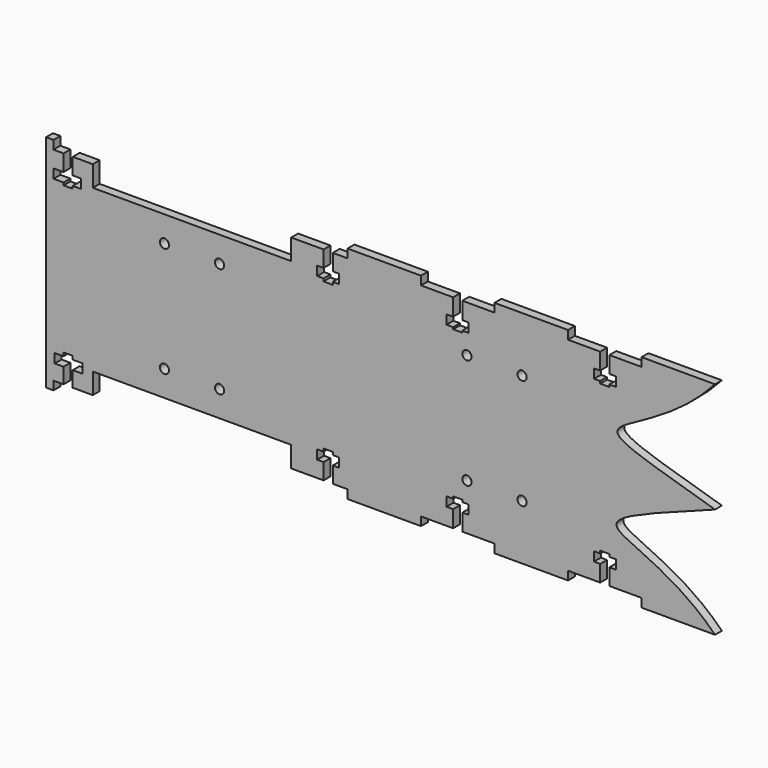
from build123d import *

# Parameters (mm, degrees)
F0_R     = 1.5875
F0_W     = 159.1020785272
F0_H     = 25.4
F1_DEPTH = 2.9718


# Not quite as in the source:
# - a feature names something its author has since deleted; it is built from what else it names


with BuildPart() as f1:
    # F0 (on Front) → F1 (new body)
    with BuildSketch(Plane.XZ):
        Polygon((-134.1324669933, 51.0296365122), (-134.1324669933, 54.0014365122), (-136.6724669933, 54.0014365122), (-136.6724669933, -22.1985634878), (-134.1324669933, -22.1985634878), (-134.1324669933, -19.2267634878), align=None)
        with BuildLine():
            Line((-130.6399669933, 51.0296365122), (-134.1324669933, 51.0296365122))
            Line((-134.1324669933, 51.0296365122), (-134.1324669933, -19.2267634878))
            Line((-134.1324669933, -19.2267634878), (-130.6399669933, -19.2267634878))
            Line((-130.6399669933, -19.2267634878), (-130.6399669933, -13.8642910361))
            Line((-130.6399669933, -13.8642910361), (-133.683725667, -13.8642910361))
            Line((-133.683725667, -13.8642910361), (-133.683725667, -10.6892910361))
            Line((-133.683725667, -10.6892910361), (-130.6399669933, -10.6892910361))
            Line((-130.6399669933, -10.6892910361), (-130.6399669933, -9.4985634878))
            Line((-130.6399669933, -9.4985634878), (-127.4649669933, -9.4985634878))
            Line((-127.4649669933, -9.4985634878), (-127.4649669933, -10.6892910361))
            Line((-127.4649669933, -10.6892910361), (-124.158725667, -10.6892910361))
            Line((-124.158725667, -10.6892910361), (-124.158725667, -13.8642910361))
            Line((-124.158725667, -13.8642910361), (-127.4649669933, -13.8642910361))
            Line((-127.4649669933, -13.8642910361), (-127.4649669933, -19.2267634878))
            Line((-127.4649669933, -19.2267634878), (-120.5434669933, -19.2267634878))
            Line((-120.5434669933, -19.2267634878), (-120.5434669933, -12.0385634878))
            Line((-120.5434669933, -12.0385634878), (-51.9634669933, -12.0385634878))
            Line((-51.9634669933, -12.0385634878), (-51.9634669933, -19.2267634878))
            Line((-51.9634669933, -19.2267634878), (-40.7874669933, -19.2267634878))
            Line((-40.7874669933, -19.2267634878), (-40.7874669933, -13.650716418))
            Line((-40.7874669933, -13.650716418), (-43.0311936414, -13.650716418))
            Line((-43.0311936414, -13.650716418), (-43.0311936414, -10.475716418))
            Line((-43.0311936414, -10.475716418), (-40.7874669933, -10.475716418))
            Line((-40.7874669933, -10.475716418), (-40.7874669933, -9.4985634878))
            Line((-40.7874669933, -9.4985634878), (-37.6124669933, -9.4985634878))
            Line((-37.6124669933, -9.4985634878), (-37.6124669933, -10.475716418))
            Line((-37.6124669933, -10.475716418), (-35.4111936414, -10.475716418))
            Line((-35.4111936414, -10.475716418), (-35.4111936414, -13.650716418))
            Line((-35.4111936414, -13.650716418), (-37.6124669933, -13.650716418))
            Line((-37.6124669933, -13.650716418), (-37.6124669933, -19.2267634878))
            Line((-37.6124669933, -19.2267634878), (-32.5324669933, -19.2267634878))
            Line((-32.5324669933, -19.2267634878), (-32.5324669933, -22.1985634878))
            Line((-32.5324669933, -22.1985634878), (-7.1324669933, -22.1985634878))
            Line((-7.1324669933, -22.1985634878), (-7.1324669933, -19.2267634878))
            Line((-7.1324669933, -19.2267634878), (3.9800330067, -19.2267634878))
            Line((3.9800330067, -19.2267634878), (3.9800330067, -13.4051909164))
            Line((3.9800330067, -13.4051909164), (1.6932926612, -13.4051909164))
            Line((1.6932926612, -13.4051909164), (1.6932926612, -10.2301909164))
            Line((1.6932926612, -10.2301909164), (3.9800330067, -10.2301909164))
            Line((3.9800330067, -10.2301909164), (3.9800330067, -9.4985634878))
            Line((3.9800330067, -9.4985634878), (7.1550330067, -9.4985634878))
            Line((7.1550330067, -9.4985634878), (7.1550330067, -10.2301909164))
            Line((7.1550330067, -10.2301909164), (9.3132926612, -10.2301909164))
            Line((9.3132926612, -10.2301909164), (9.3132926612, -13.4051909164))
            Line((9.3132926612, -13.4051909164), (7.1550330067, -13.4051909164))
            Line((7.1550330067, -13.4051909164), (7.1550330067, -19.2267634878))
            Line((7.1550330067, -19.2267634878), (18.2675330067, -19.2267634878))
            Line((18.2675330067, -19.2267634878), (18.2675330067, -22.1985634878))
            Line((18.2675330067, -22.1985634878), (43.6675330067, -22.1985634878))
            Line((43.6675330067, -22.1985634878), (43.6675330067, -19.2267634878))
            Line((43.6675330067, -19.2267634878), (54.7800330067, -19.2267634878))
            Line((54.7800330067, -19.2267634878), (54.7800330067, -13.545062393))
            Line((54.7800330067, -13.545062393), (52.6228938252, -13.545062393))
            Line((52.6228938252, -13.545062393), (52.6228938252, -10.370062393))
            Line((52.6228938252, -10.370062393), (54.7800330067, -10.370062393))
            Line((54.7800330067, -10.370062393), (54.7800330067, -9.4985634878))
            Line((54.7800330067, -9.4985634878), (57.9550330067, -9.4985634878))
            Line((57.9550330067, -9.4985634878), (57.9550330067, -10.370062393))
            Line((57.9550330067, -10.370062393), (60.2428938252, -10.370062393))
            Line((60.2428938252, -10.370062393), (60.2428938252, -13.545062393))
            Line((60.2428938252, -13.545062393), (57.9550330067, -13.545062393))
            Line((57.9550330067, -13.545062393), (57.9550330067, -19.2267634878))
            Line((57.9550330067, -19.2267634878), (69.0675330067, -19.2267634878))
            Line((69.0675330067, -19.2267634878), (69.0675330067, -22.1985634878))
            Line((69.0675330067, -22.1985634878), (94.4675330067, -22.1985634878))
            add(Edge.make_bspline(
                [(94.4675330067, 15.9014365122), (33.4221309805, -6.5926179945), (67.8742191577, 4.6496394366), (94.4675330067, -22.1985634878)],
                knots=[0, 0, 0, 0, 38.1, 38.1, 38.1, 38.1], degree=3))
            add(Edge.make_bspline(
                [(94.4675330067, 54.0014365122), (67.8547954941, 24.2413681328), (34.147437551, 33.6619180903), (94.4675330067, 15.9014365122)],
                knots=[0, 0, 0, 0, 38.1, 38.1, 38.1, 38.1], degree=3))
            Line((94.4675330067, 54.0014365122), (69.0675330067, 54.0014365122))
            Line((69.0675330067, 54.0014365122), (69.0675330067, 51.0296365122))
            Line((69.0675330067, 51.0296365122), (57.9550330067, 51.0296365122))
            Line((57.9550330067, 51.0296365122), (57.9550330067, 45.263365978))
            Line((57.9550330067, 45.263365978), (60.3188354051, 45.263365978))
            Line((60.3188354051, 45.263365978), (60.3188354051, 42.088365978))
            Line((60.3188354051, 42.088365978), (57.9550330067, 42.088365978))
            Line((57.9550330067, 42.088365978), (57.9550330067, 41.3014365122))
            Line((57.9550330067, 41.3014365122), (54.7800330067, 41.3014365122))
            Line((54.7800330067, 41.3014365122), (54.7800330067, 42.088365978))
            Line((54.7800330067, 42.088365978), (52.6988354051, 42.088365978))
            Line((52.6988354051, 42.088365978), (52.6988354051, 45.263365978))
            Line((52.6988354051, 45.263365978), (54.7800330067, 45.263365978))
            Line((54.7800330067, 45.263365978), (54.7800330067, 51.0296365122))
            Line((54.7800330067, 51.0296365122), (43.6675330067, 51.0296365122))
            Line((43.6675330067, 51.0296365122), (43.6675330067, 54.0014365122))
            Line((43.6675330067, 54.0014365122), (18.2675330067, 54.0014365122))
            Line((18.2675330067, 54.0014365122), (18.2675330067, 51.0296365122))
            Line((18.2675330067, 51.0296365122), (7.1550330067, 51.0296365122))
            Line((7.1550330067, 51.0296365122), (7.1550330067, 45.1199758291))
            Line((7.1550330067, 45.1199758291), (9.3046905002, 45.1199758291))
            Line((9.3046905002, 45.1199758291), (9.3046905002, 41.9449758291))
            Line((9.3046905002, 41.9449758291), (7.1550330067, 41.9449758291))
            Line((7.1550330067, 41.9449758291), (7.1550330067, 41.3014365122))
            Line((7.1550330067, 41.3014365122), (3.9800330067, 41.3014365122))
            Line((3.9800330067, 41.3014365122), (3.9800330067, 41.9449758291))
            Line((3.9800330067, 41.9449758291), (1.6846905002, 41.9449758291))
            Line((1.6846905002, 41.9449758291), (1.6846905002, 45.1199758291))
            Line((1.6846905002, 45.1199758291), (3.9800330067, 45.1199758291))
            Line((3.9800330067, 45.1199758291), (3.9800330067, 51.0296365122))
            Line((3.9800330067, 51.0296365122), (-7.1324669933, 51.0296365122))
            Line((-7.1324669933, 51.0296365122), (-7.1324669933, 54.0014365122))
            Line((-7.1324669933, 54.0014365122), (-32.5324669933, 54.0014365122))
            Line((-32.5324669933, 54.0014365122), (-32.5324669933, 51.0296365122))
            Line((-32.5324669933, 51.0296365122), (-37.6124669933, 51.0296365122))
            Line((-37.6124669933, 51.0296365122), (-37.6124669933, 45.4024068505))
            Line((-37.6124669933, 45.4024068505), (-35.3795323992, 45.4024068505))
            Line((-35.3795323992, 45.4024068505), (-35.3795323992, 42.2274068505))
            Line((-35.3795323992, 42.2274068505), (-37.6124669933, 42.2274068505))
            Line((-37.6124669933, 42.2274068505), (-37.6124669933, 41.3014365122))
            Line((-37.6124669933, 41.3014365122), (-40.7874669933, 41.3014365122))
            Line((-40.7874669933, 41.3014365122), (-40.7874669933, 42.2274068505))
            Line((-40.7874669933, 42.2274068505), (-42.9995323992, 42.2274068505))
            Line((-42.9995323992, 42.2274068505), (-42.9995323992, 45.4024068505))
            Line((-42.9995323992, 45.4024068505), (-40.7874669933, 45.4024068505))
            Line((-40.7874669933, 45.4024068505), (-40.7874669933, 51.0296365122))
            Line((-40.7874669933, 51.0296365122), (-51.9634669933, 51.0296365122))
            Line((-51.9634669933, 51.0296365122), (-51.9634669933, 43.8414365122))
            Line((-51.9634669933, 43.8414365122), (-120.5434669933, 43.8414365122))
            Line((-120.5434669933, 43.8414365122), (-120.5434669933, 51.0296365122))
            Line((-120.5434669933, 51.0296365122), (-127.4649669933, 51.0296365122))
            Line((-127.4649669933, 51.0296365122), (-127.4649669933, 45.3533373266))
            Line((-127.4649669933, 45.3533373266), (-124.5652367949, 45.3533373266))
            Line((-124.5652367949, 45.3533373266), (-124.5652367949, 42.1783373266))
            Line((-124.5652367949, 42.1783373266), (-127.4649669933, 42.1783373266))
            Line((-127.4649669933, 42.1783373266), (-127.4649669933, 41.3014365122))
            Line((-127.4649669933, 41.3014365122), (-130.6399669933, 41.3014365122))
            Line((-130.6399669933, 41.3014365122), (-130.6399669933, 42.1783373266))
            Line((-130.6399669933, 42.1783373266), (-134.0902367949, 42.1783373266))
            Line((-134.0902367949, 42.1783373266), (-134.0902367949, 45.3533373266))
            Line((-134.0902367949, 45.3533373266), (-130.6399669933, 45.3533373266))
            Line((-130.6399669933, 45.3533373266), (-130.6399669933, 51.0296365122))
        make_face()
        with Locations((-95.7784669933, -3.1485634878)):
            Circle(F0_R, mode=Mode.SUBTRACT)
        with BuildLine():
            ThreePointArc((-75.1409669933, -3.1485634878), (-76.7284669933, -4.7360634878), (-78.3159669933, -3.1485634878))
            ThreePointArc((-78.3159669933, -3.1485634878), (-76.7284669933, -1.5610634878), (-75.1409669933, -3.1485634878))
        make_face(mode=Mode.SUBTRACT)
        with Locations((8.7425330067, -3.1485634878)):
            Circle(F0_R, mode=Mode.SUBTRACT)
        with BuildLine():
            ThreePointArc((29.3800330067, -3.1485634878), (27.7925330067, -4.7360634878), (26.2050330067, -3.1485634878))
            ThreePointArc((26.2050330067, -3.1485634878), (27.7925330067, -1.5610634878), (29.3800330067, -3.1485634878))
        make_face(mode=Mode.SUBTRACT)
        with Locations((-29.1814277297, 15.9014365122)):
            Rectangle(F0_W, F0_H, mode=Mode.SUBTRACT)
        with Locations((-95.7784669933, 34.9514365122)):
            Circle(F0_R, mode=Mode.SUBTRACT)
        with BuildLine():
            ThreePointArc((-75.1409669933, 34.9514365122), (-76.7284669933, 33.3639365122), (-78.3159669933, 34.9514365122))
            ThreePointArc((-78.3159669933, 34.9514365122), (-76.7284669933, 36.5389365122), (-75.1409669933, 34.9514365122))
        make_face(mode=Mode.SUBTRACT)
        with Locations((8.7425330067, 34.9514365122)):
            Circle(F0_R, mode=Mode.SUBTRACT)
        with BuildLine():
            ThreePointArc((29.3800330067, 34.9514365122), (27.7925330067, 33.3639365122), (26.2050330067, 34.9514365122))
            ThreePointArc((26.2050330067, 34.9514365122), (27.7925330067, 36.5389365122), (29.3800330067, 34.9514365122))
        make_face(mode=Mode.SUBTRACT)
        with Locations((-29.1814277297, 15.9014365122)):
            Rectangle(F0_W, F0_H)
    extrude(amount=F1_DEPTH)


solid = f1.part
